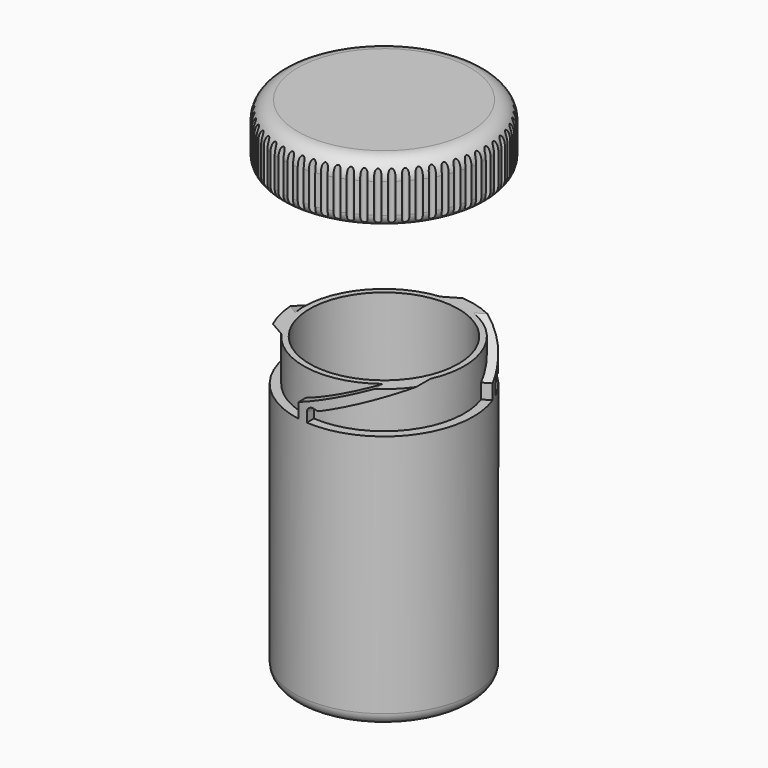
from build123d import *

# Parameters (mm, degrees)
F0_R             = 15
F1_DEPTH         = 50
F2_R             = 2
F3_R             = 16.5
F3_R_2           = 13.5
F4_DEPTH         = 7
F6_DEPTH         = 16
F6_COPIES_COUNT  = 3
F8_R             = 22.5
F8_R_2           = 15
F9_DEPTH         = 7
F11_R            = 17.5
F12_DEPTH        = 10
F13_R            = 3
F14_R            = 2
F15_R            = 0.5
F16_DEPTH        = 10
F16_COPIES_COUNT = 60
F17_R            = 15
F18_DEPTH        = 7
F19_R            = 0.5
F20_DEPTH        = 16
F20_COPIES_COUNT = 3
F22_R            = 13.75
F23_DEPTH        = 7
F24_R            = 12.5
F25_DEPTH        = 47


# Not quite as in the source:
# - a pattern or mirror of a feature is missing from the dataset's text; its kind, count and spacing are read off the source's solid


with BuildPart() as f1:
    # F0 (on Top) → F1 (new body)
    with BuildSketch(Plane.XY):
        Circle(F0_R)
    extrude(amount=F1_DEPTH)

    # F2
    f2_edges = [f1.edges().sort_by_distance(p)[0] for p in [
        (-15, 0, 0),
    ]]
    fillet(f2_edges, radius=F2_R)

    # F3 (on face) → F4 (cut)
    with BuildSketch(Plane.XY.offset(50)):
        Circle(F3_R)
        Circle(F3_R_2, mode=Mode.SUBTRACT)
    extrude(amount=-F4_DEPTH, mode=Mode.SUBTRACT)

    # F5 (on Front) → F6 (join)
    with BuildSketch(Plane.XZ):
        with BuildLine():
            Line((1.1912623771, 45.4053826384), (12.2836499253, 50))
            Line((12.2836499253, 50), (8.3639610307, 50))
            Line((8.3639610307, 50), (-2.5, 45.5))
            Line((-2.5, 45.5), (-2.5, 43))
            Line((-2.5, 43), (-1, 43))
            Line((-1, 43), (-1, 44.5))
            ThreePointArc((-1, 44.5), (-0.5457611784, 45.3379407713), (0.4042894724, 45.4146310855))
            ThreePointArc((0.4042894724, 45.4146310855), (0.7968278306, 45.3293312177), (1.1912623771, 45.4053826384))
        make_face()
    f6 = extrude(amount=F6_DEPTH)

    # F6_copies: F6 ×3 about axis
    f6_copies_axis = Axis((0, 0, 0), (0, 0, 1))
    for i in range(1, F6_COPIES_COUNT):
        add(f6.rotate(f6_copies_axis, i * 360 / F6_COPIES_COUNT))

    # F8 (on face) → F9 (cut)
    with BuildSketch(Plane.XY.offset(50)):
        Circle(F8_R)
        Circle(F8_R_2, mode=Mode.SUBTRACT)
    extrude(amount=-F9_DEPTH, mode=Mode.SUBTRACT)

    # F24 (on face) → F25 (cut)
    with BuildSketch(Plane.XY.offset(50)):
        Circle(F24_R)
    extrude(amount=-F25_DEPTH, mode=Mode.SUBTRACT)


with BuildPart() as f12:
    # F11 (on face) → F12 (new body)
    with BuildSketch(Plane.XY.offset(75)):
        Circle(F11_R)
    extrude(amount=F12_DEPTH)

    # F13
    f13_edges = [f12.edges().sort_by_distance(p)[0] for p in [
        (-17.5, 0, 85),
    ]]
    fillet(f13_edges, radius=F13_R)

    # F14
    f14_edges = [f12.edges().sort_by_distance(p)[0] for p in [
        (-17.5, 0, 75),
    ]]
    fillet(f14_edges, radius=F14_R)

    # F15 (on face) → F16 (cut)
    with BuildSketch(Plane.XY.offset(85)):
        with Locations((17.5, 0)):
            Circle(F15_R)
    f16 = extrude(amount=-F16_DEPTH, mode=Mode.SUBTRACT)

    # F16_copies: F16 ×60 about axis
    f16_copies_axis = Axis((0, 0, 0), (0, 0, 1))
    for i in range(1, F16_COPIES_COUNT):
        add(f16.rotate(f16_copies_axis, i * 360 / F16_COPIES_COUNT), mode=Mode.SUBTRACT)

    # F17 (on face) → F18 (cut)
    with BuildSketch(Plane(origin=(0, 0, 75), x_dir=(1, 0, 0), z_dir=(0, 0, -1))):
        Circle(F17_R)
    extrude(amount=-F18_DEPTH, mode=Mode.SUBTRACT)

    # F19 (on Right) → F20 (join)
    with BuildSketch(Plane.YZ):
        with Locations((0, 76)):
            Circle(F19_R)
    f20 = extrude(amount=F20_DEPTH)

    # F20_copies: F20 ×3 about axis
    f20_copies_axis = Axis((0, 0, 0), (0, 0, 1))
    for i in range(1, F20_COPIES_COUNT):
        add(f20.rotate(f20_copies_axis, i * 360 / F20_COPIES_COUNT))

    # F22 (on face) → F23 (cut)
    with BuildSketch(Plane(origin=(0, 0, 75), x_dir=(1, 0, 0), z_dir=(0, 0, -1))):
        Circle(F22_R)
    extrude(amount=-F23_DEPTH, mode=Mode.SUBTRACT)


solid = Compound([f1.part, f12.part])
